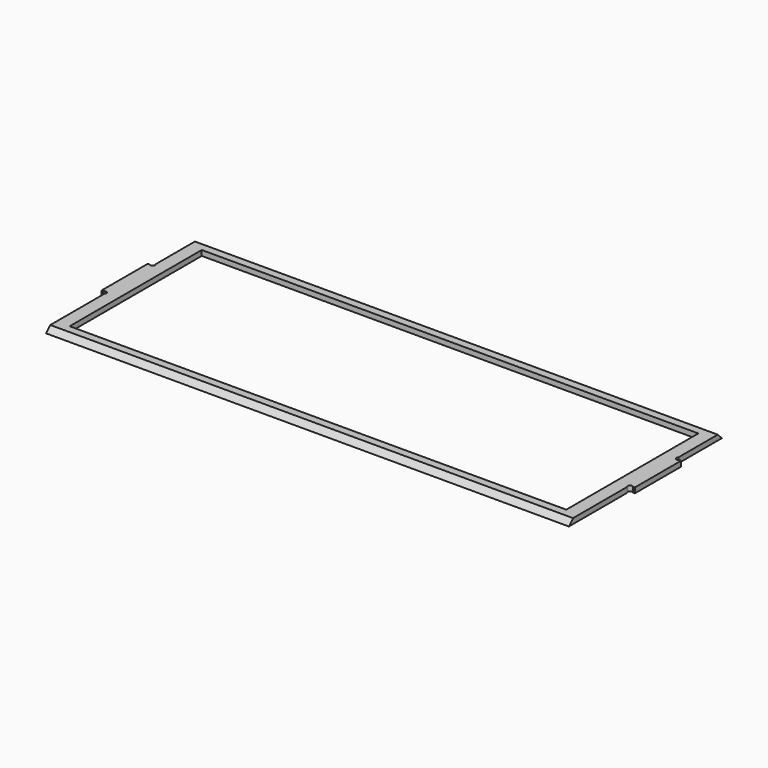
from build123d import *

# Parameters (mm, degrees)
F0_W     = 189.5
F0_H     = 63
F1_DEPTH = 2
F2_SIZE  = 1.99999
F3_SIZE  = 1.99999


# Not quite as in the source:
# - a fillet or chamfer is up to 0.001 mm smaller than in the source, because OpenCascade refuses the exact size


with BuildPart() as f1:
    # F0 (on Top) → F1 (new body)
    with BuildSketch(Plane.XY):
        with BuildLine():
            Line((-99.2, 51), (-100, 51))
            Line((-100, 51), (-100, 29))
            Line((-100, 29), (-99.2, 29))
            ThreePointArc((-99.2, 29), (-98, 29), (-98, 27.8))
            Line((-98, 27.8), (-98, 0))
            Line((-98, 0), (101.5, 0))
            Line((101.5, 0), (101.5, 27.8))
            ThreePointArc((101.5, 27.8), (101.5, 29), (102.7, 29))
            Line((102.7, 29), (103.5, 29))
            Line((103.5, 29), (103.5, 51))
            Line((103.5, 51), (102.7, 51))
            ThreePointArc((102.7, 51), (101.5, 51), (101.5, 52.2))
            Line((101.5, 52.2), (101.5, 73))
            Line((101.5, 73), (-98, 73))
            Line((-98, 73), (-98, 52.2))
            ThreePointArc((-98, 52.2), (-98, 51), (-99.2, 51))
        make_face()
        with Locations((1.75, 36.5)):
            Rectangle(F0_W, F0_H, mode=Mode.SUBTRACT)
    extrude(amount=F1_DEPTH)

    # F2 (size 2 in the source; OpenCascade refuses exactly that, so slightly less here)
    f2_edges = [f1.edges().sort_by_distance(p)[0] for p in [
        (1.75, 0, 2),
    ]]
    chamfer(f2_edges, length=F2_SIZE)

    # F3 (size 2 in the source; OpenCascade refuses exactly that, so slightly less here)
    f3_edges = [f1.edges().sort_by_distance(p)[0] for p in [
        (1.75, 73, 2),
    ]]
    chamfer(f3_edges, length=F3_SIZE)


solid = f1.part
